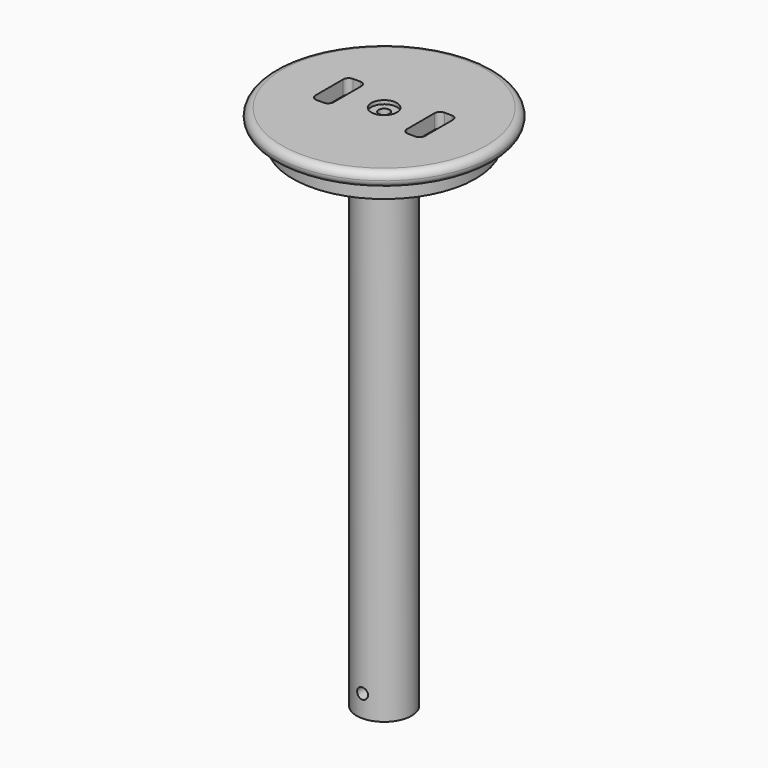
from build123d import *

# Parameters (mm, degrees)
F0_R          = 7.5
F1_DEPTH      = 135
F2_R          = 25
F3_DEPTH      = 5
F4_R          = 1.5
F5_DEPTH      = 7.5
F5_DEPTH_BACK = 7.5
F6_R          = 2
F7_DEPTH      = 10
F8_R          = 30
F8_R_2        = 2
F9_DEPTH      = 4
F11_DEPTH     = 4
F12_R         = 2
F12_R_2       = 1.5
F13_DEPTH     = 4
F12_R_3       = 3.5
F14_DEPTH     = 1
F15_R         = 1.99999


# Not quite as in the source:
# - a fillet or chamfer is up to 0.001 mm smaller than in the source, because OpenCascade refuses the exact size


with BuildPart() as f1:
    # F0 (on Top) → F1 (new body)
    with BuildSketch(Plane.XY):
        Circle(F0_R)
    extrude(amount=F1_DEPTH)

    # F2 (on face) → F3 (join)
    with BuildSketch(Plane.XY.offset(135)):
        Circle(F2_R)
    extrude(amount=F3_DEPTH)

    # F4 (on Front) → F5 (cut, two sides)
    with BuildSketch(Plane.XZ) as f5_sk:
        with Locations((0, 6)):
            Circle(F4_R)
    extrude(amount=-F5_DEPTH, mode=Mode.SUBTRACT)
    extrude(f5_sk.sketch, amount=F5_DEPTH_BACK, mode=Mode.SUBTRACT)

    # F6 (on face) → F7 (cut)
    with BuildSketch(Plane.XY.offset(140)):
        Circle(F6_R)
    extrude(amount=-F7_DEPTH, mode=Mode.SUBTRACT)


with BuildPart() as f9:
    # F8 (on face) → F9 (new body)
    with BuildSketch(Plane.XY.offset(140)):
        Circle(F8_R)
        Circle(F8_R_2, mode=Mode.SUBTRACT)
    extrude(amount=F9_DEPTH)

    # F10 (on face) → F11 (cut, through all)
    with BuildSketch(Plane.XY.offset(144)):
        with BuildLine():
            Line((13.5, 6.25), (11.5, 6.25))
            ThreePointArc((11.5, 6.25), (10.4393398282, 5.8106601718), (10, 4.75))
            Line((10, 4.75), (10, -4.75))
            ThreePointArc((10, -4.75), (10.4393398282, -5.8106601718), (11.5, -6.25))
            Line((11.5, -6.25), (13.5, -6.25))
            ThreePointArc((13.5, -6.25), (14.5606601718, -5.8106601718), (15, -4.75))
            Line((15, -4.75), (15, 4.75))
            ThreePointArc((15, 4.75), (14.5606601718, 5.8106601718), (13.5, 6.25))
        make_face()
        with BuildLine():
            ThreePointArc((-10, 4.75), (-10.4393398282, 5.8106601718), (-11.5, 6.25))
            Line((-11.5, 6.25), (-13.5, 6.25))
            ThreePointArc((-13.5, 6.25), (-14.5606601718, 5.8106601718), (-15, 4.75))
            Line((-15, 4.75), (-15, -4.75))
            ThreePointArc((-15, -4.75), (-14.5606601718, -5.8106601718), (-13.5, -6.25))
            Line((-13.5, -6.25), (-11.5, -6.25))
            ThreePointArc((-11.5, -6.25), (-10.4393398282, -5.8106601718), (-10, -4.75))
            Line((-10, -4.75), (-10, 4.75))
        make_face()
    extrude(amount=-F11_DEPTH, mode=Mode.SUBTRACT)

    # F12 (on face) → F13 (join, through all)
    with BuildSketch(Plane.XY.offset(144)):
        Circle(F12_R)
        Circle(F12_R_2, mode=Mode.SUBTRACT)
    extrude(amount=-F13_DEPTH)

    # F12 (on face) → F14 (cut)
    with BuildSketch(Plane.XY.offset(144)):
        Circle(F12_R_3)
        Circle(F12_R, mode=Mode.SUBTRACT)
        Circle(F12_R)
        Circle(F12_R_2, mode=Mode.SUBTRACT)
    extrude(amount=-F14_DEPTH, mode=Mode.SUBTRACT)

    # F15 (radius 2 in the source; OpenCascade refuses exactly that, so slightly less here)
    f15_edges = [f9.edges().sort_by_distance(p)[0] for p in [
        (-30, 0, 144),
        (-30, 0, 140),
    ]]
    fillet(f15_edges, radius=F15_R)


solid = Compound([f1.part, f9.part])
